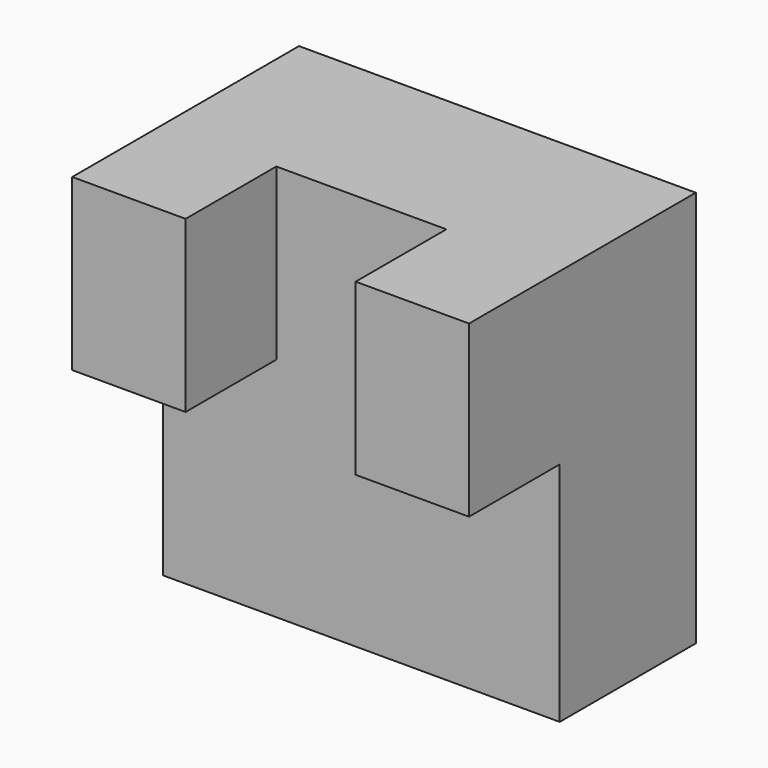
from build123d import *

# Parameters (mm, degrees)
F0_W     = 177.8
F0_H     = 177.8
F1_DEPTH = 50.8
F2_DEPTH = 25.4
F3_W     = 50.8
F3_H     = 76.2
F4_DEPTH = 50.8


# Not quite as in the source:
# - a feature names something its author has since deleted; it is built from what else it names


with BuildPart() as f1:
    # F0 (on Front) → F1 (new body)
    with BuildSketch(Plane.XZ):
        with Locations((0.9207129478, 25.5247855931)):
            Rectangle(F0_W, F0_H)
    extrude(amount=F1_DEPTH)

    # F2 (add, symmetric): a face of the model
    f2_faces = [f1.faces().sort_by_distance(p)[0] for p in [
        (0.9207129478, -50.8, 25.5247855931),
    ]]
    extrude(f2_faces, amount=F2_DEPTH, both=True)

    # F3 (on face) → F4 (join)
    with BuildSketch(Plane.XZ.offset(76.2)):
        with Locations((-62.5792870522, 76.3247855931)):
            Rectangle(F3_W, F3_H)
        with Locations((64.4207129478, 76.3247855931)):
            Rectangle(F3_W, F3_H)
    extrude(amount=F4_DEPTH)


solid = f1.part
